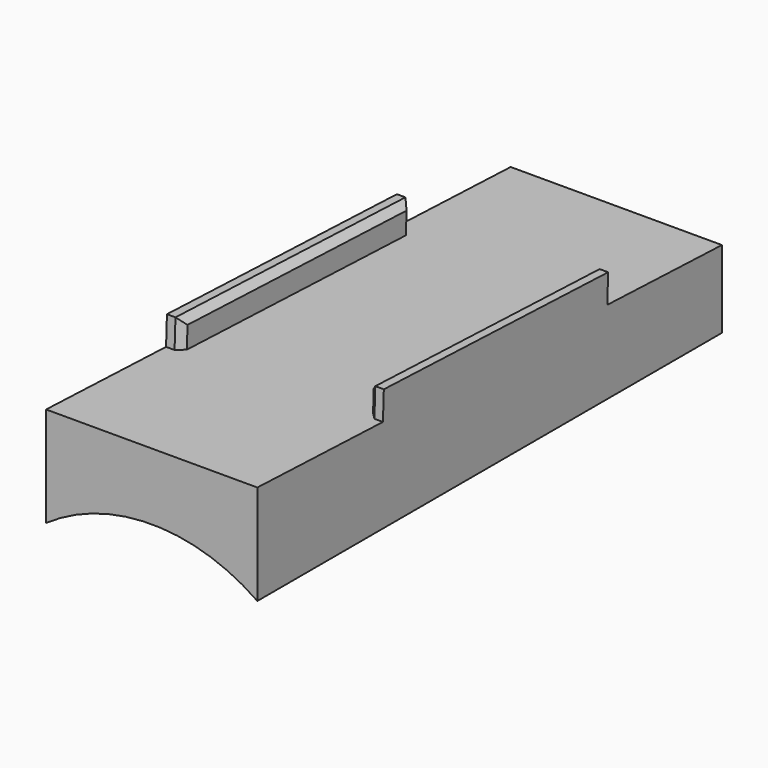
from build123d import *

# Parameters (mm, degrees)
F1_DEPTH = 30.97
F2_W     = 2.25
F2_H     = 41.1360506777
F2_H_2   = 42.1689638739
F3_DEPTH = 4.15
F4_SIZE  = 1
F5_SIZE  = 1
F7_DEPTH = 85.13


with BuildPart() as f1:
    # F0 (on Right) → F1 (new body)
    with BuildSketch(Plane.YZ):
        Polygon((97.6600019388, 28.3032343221), (97.6600019388, 34.6382343221), (12.5300019388, 37.9532343221), (12.5300019388, 28.3032343221), align=None)
    extrude(amount=-F1_DEPTH)

    # F2 (on face) → F3 (join)
    with BuildSketch(Plane(origin=(0, 1.4946493439, 38.3829558521), x_dir=(1, 0, 0), z_dir=(0, 0.0389109537, 0.9992426821))):
        with Locations((-1.125, 54.6446547341)):
            Rectangle(F2_W, F2_H)
        with Locations((-29.845, 54.128198136)):
            Rectangle(F2_W, F2_H_2)
    extrude(amount=F3_DEPTH)

    # F4
    f4_edges = [f1.edges().sort_by_distance(p)[0] for p in [
        (-28.72, 55.743336, 40.423633),
        (-2.25, 56.259401, 40.403537),
    ]]
    chamfer(f4_edges, length=F4_SIZE)

    # F5
    f5_edges = [f1.edges().sort_by_distance(p)[0] for p in [
        (-2.25, 76.711654, 37.030166),
        (-2.25, 35.606757, 38.630809),
        (-28.72, 34.574626, 38.671001),
        (-28.72, 76.711654, 37.030166),
    ]]
    chamfer(f5_edges, length=F5_SIZE)

    # F6 (on face) → F7 (join, through all)
    with BuildSketch(Plane.XZ.offset(-12.5300019388)):
        with BuildLine():
            Line((0, 28.3032343221), (-30.97, 28.3032343221))
            Line((-30.97, 28.3032343221), (-30.97, 23.3032343221))
            ThreePointArc((-30.97, 23.3032343221), (-15.485, 28.1745693779), (0, 23.3032343221))
            Line((0, 23.3032343221), (0, 28.3032343221))
        make_face()
    extrude(amount=-F7_DEPTH)


solid = f1.part
